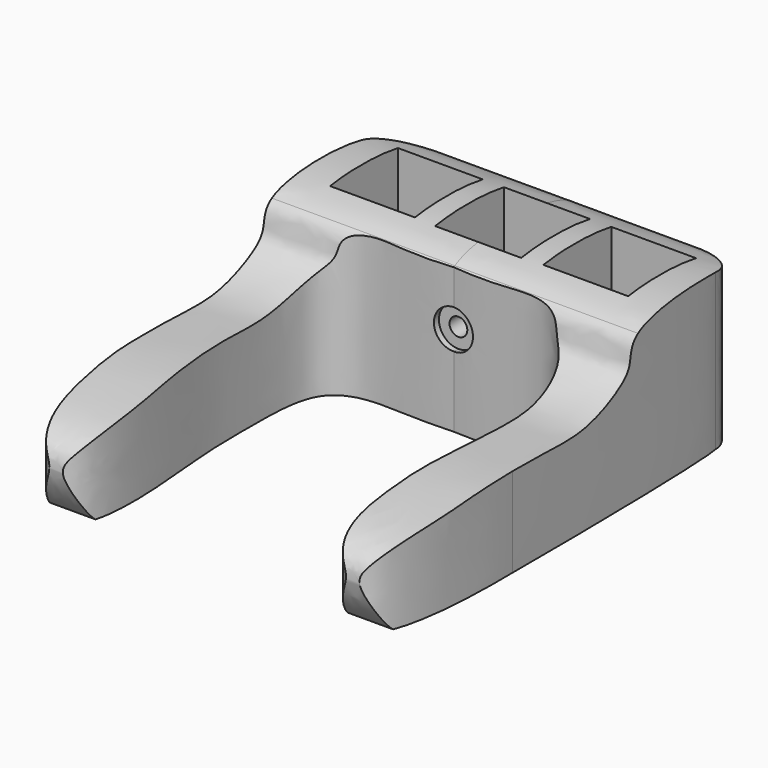
from build123d import *

# Parameters (mm, degrees)
F0_W      = 20
F0_H      = 20
F0_W_2    = 20.3
F0_H_2    = 20.3
F1_DEPTH  = 42
F2_DEPTH  = 5
F4_DEPTH  = 50.2
F7_D      = 4.2
F8_DEPTH  = 2
F10_R     = 4.6
F10_R_2   = 2.1
F11_DEPTH = 3


with BuildPart() as f1:
    # F0 (on Top) → F1 (new body)
    with BuildSketch(Plane.XY):
        with BuildLine():
            add(Edge.make_bspline(
                [(-41.9893918588, 45.2532443083), (-41.5805276857, 63.0376977926), (41.5805276857, 63.0376977926), (41.9893918588, 45.2532443083)],
                knots=[0, 0, 0, 0, 83.9787837175, 83.9787837175, 83.9787837175, 83.9787837175], degree=3))
            add(Edge.make_bspline(
                [(-41.9893918588, 45.2532443083), (-43.034663613, 39.9344238318), (-43.5955785215, 5.4338923655), (-43.5178056359, -16.4565779269)],
                knots=[0, 0, 0, 0, 61.7287470225, 61.7287470225, 61.7287470225, 61.7287470225], degree=3))
            add(Edge.make_bspline(
                [(0, 20.6839926541), (-2.6962849926, 20.5284869173), (-11.5189399188, 20.388587782), (-20.4666045121, 21.273432606), (-30.5925904183, 17.3737690184), (-30.5124516546, -1.6110444599), (-30.8051000661, -15.4807460819), (-25.9776494371, -52.8874219866), (-43.3534468321, -54.8813612045), (-43.7026559925, -25.5815181898), (-43.5178056359, -16.4565779269)],
                knots=[0, 0, 0, 0, 0.1041048083, 0.2004631786, 0.2927409852, 0.4187580647, 0.5483414857, 0.729234525, 0.8146025633, 1, 1, 1, 1], degree=3))
            add(Edge.make_bspline(
                [(0, 20.6839926541), (2.6962849926, 20.5284869173), (11.5189399188, 20.388587782), (20.4666045121, 21.273432606), (30.5925904183, 17.3737690184), (30.5124516546, -1.6110444599), (30.8051000661, -15.4807460819), (25.9776494371, -52.8874219866), (43.3534468321, -54.8813612045), (43.7026559925, -25.5815181898), (43.5178056359, -16.4565779269)],
                knots=[0, 0, 0, 0, 0.1041048083, 0.2004631786, 0.2927409852, 0.4187580647, 0.5483414857, 0.729234525, 0.8146025633, 1, 1, 1, 1], degree=3))
            add(Edge.make_bspline(
                [(41.9893918588, 45.2532443083), (43.034663613, 39.9344238318), (43.5955785215, 5.4338923655), (43.5178056359, -16.4565779269)],
                knots=[0, 0, 0, 0, 61.7287470225, 61.7287470225, 61.7287470225, 61.7287470225], degree=3))
        make_face()
        with Locations((-25.15, 38.1104509056)):
            Rectangle(F0_W, F0_H, mode=Mode.SUBTRACT)
        with Locations((0, 37.9604509056)):
            Rectangle(F0_W_2, F0_H_2, mode=Mode.SUBTRACT)
        with Locations((25.15, 38.1104509056)):
            Rectangle(F0_W, F0_H, mode=Mode.SUBTRACT)
    extrude(amount=F1_DEPTH)

    # F0 (on Top) → F2 (join)
    with BuildSketch(Plane.XY):
        with Locations((-25.15, 38.1104509056)):
            Rectangle(F0_W, F0_H)
        with Locations((25.15, 38.1104509056)):
            Rectangle(F0_W, F0_H)
        with Locations((0, 37.9604509056)):
            Rectangle(F0_W_2, F0_H_2)
    extrude(amount=F2_DEPTH)

    # F3 (on Right) → F4 (intersect, symmetric)
    with BuildSketch(Plane.YZ):
        with BuildLine():
            add(Edge.make_bspline(
                [(-47.8295497596, 0), (-49.7771650798, 1.6648228017), (-58.8353398265, 16.0825952246), (-36.053518274, 19.4445651222), (-29.1423114031, 20.4311252049), (-22.6595967581, 21.0747628797), (-7.9374673338, 21.1911129955), (4.9260518726, 20.2077119282), (15.2290319706, 24.7859534705), (19.1990347429, 28.5312082845), (18.5675170217, 32.7625981001), (20.9730211645, 34.3544632196)],
                knots=[0, 0, 0, 0, 0.0822439151, 0.1758372267, 0.2383560063, 0.293613831, 0.3794539338, 0.4622157247, 0.535609697, 0.5847542789, 0.6400956608, 0.6400956608, 0.6400956608, 0.6400956608], degree=3))
            Line((-47.8295497596, 0), (54.7501146793, 0))
            add(Edge.make_bspline(
                [(54.3967820704, 34.3544632196), (58.3514929801, 32.1724468284), (57.6038308679, 24.3825431975), (59.6783683255, 8.3854050639), (55.4016424787, 1.6173290669), (54.7501146793, 0)],
                knots=[0.7699169117, 0.7699169117, 0.7699169117, 0.7699169117, 0.8426363761, 0.9338830654, 1, 1, 1, 1], degree=3))
            Line((54.3967820704, 34.3544632196), (20.9730211645, 34.3544632196))
        make_face()
        with BuildLine():
            add(Edge.make_bspline(
                [(20.9730211645, 34.3544632196), (26.6159152585, 38.0887017608), (47.3366982021, 38.2498727897), (54.3967820704, 34.3544632196)],
                knots=[0.6400956608, 0.6400956608, 0.6400956608, 0.6400956608, 0.7699169117, 0.7699169117, 0.7699169117, 0.7699169117], degree=3))
            Line((20.9730211645, 34.3544632196), (54.3967820704, 34.3544632196))
        make_face()
    extrude(amount=F4_DEPTH, both=True, mode=Mode.INTERSECT)

    # F7 (through all)
    with Locations(Plane.XZ.offset(-20)):
        with Locations((0, 21.2752800435)):
            Hole(F7_D / 2)

    # F6 (on offset) → F8 (cut)
    with BuildSketch(Plane.XZ.offset(-20)):
        with BuildLine():
            ThreePointArc((4.6, 21.2752800435), (3.2526911935, 24.5279712369), (0, 25.8752800435))
            Line((0, 25.8752800435), (0, 16.6752800435))
            ThreePointArc((0, 16.6752800435), (3.2526911935, 18.02258885), (4.6, 21.2752800435))
        make_face()
        with BuildLine():
            Line((0, 16.6752800435), (0, 25.8752800435))
            ThreePointArc((0, 25.8752800435), (-4.6, 21.2752800435), (0, 16.6752800435))
        make_face()
    extrude(amount=-F8_DEPTH, mode=Mode.SUBTRACT)

    # F10 (on offset) → F11 (cut)
    with BuildSketch(Plane.XZ.offset(-60)):
        with Locations((0, 21.2752800435)):
            Circle(F10_R)
        with Locations((0, 21.2752800435)):
            Circle(F10_R_2, mode=Mode.SUBTRACT)
    extrude(amount=F11_DEPTH, mode=Mode.SUBTRACT)


solid = f1.part
